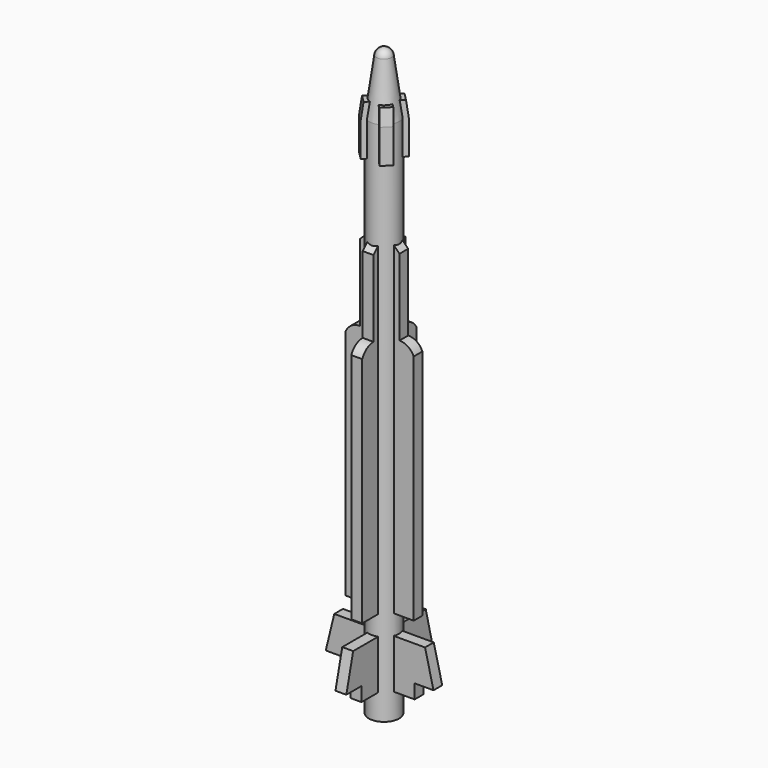
from build123d import *

# Parameters (mm, degrees)
F3_DEPTH     = 0.2
F6_DEPTH     = 0.2
F7_COUNT     = 4
F8_T4_DEPTH  = 1.685841494
F8_S5_R      = 0.5555555556
F8_T6_DEPTH  = 2
F8_T10_DEPTH = 1.685841494
F8_S11_R     = 0.5555555556
F8_T12_DEPTH = 2
F8_T16_DEPTH = 1.685841494
F8_S17_R     = 0.5555555556
F8_T18_DEPTH = 2
F8_T22_DEPTH = 1.685841494
F8_S23_R     = 0.5555555556
F8_T24_DEPTH = 2


# Not quite as in the source:
# - a fillet or chamfer that OpenCascade refuses, or shapes differently, is made with other operations: its cross-section is extruded or revolved along the edge and cut away or added
# - a feature names something its author has since deleted; it is built from what else it names


with BuildPart() as f1:
    # F0 (on Front) → F1 (revolve)
    with BuildSketch(Plane.XZ):
        with BuildLine():
            Line((0, 21.5277777778), (0, 0))
            Line((0, 0), (0.5555555556, 0))
            Line((0.5555555556, 0), (0.5555555556, 19.3055555556))
            Line((0.5555555556, 19.3055555556), (0.2793333296, 21.2847222222))
            ThreePointArc((0.2793333296, 21.2847222222), (0.185137187, 21.4585073218), (0, 21.5277777778))
        make_face()
    revolve(axis=Axis((0, 0, 10.7638888889), (0, 0, 1)))

    # F2 (on Front) → F3 (join, symmetric)
    with BuildSketch(Plane.XZ):
        with BuildLine():
            Line((0, 15.4166666667), (0, 3.4722222222))
            Line((0, 3.4722222222), (1.25, 3.4722222222))
            Line((1.25, 3.4722222222), (1.25, 12.0138888889))
            ThreePointArc((1.25, 12.0138888889), (1.0421485482, 12.2663478223), (0.7291666667, 12.3611111111))
            Line((0.7291666667, 12.3611111111), (0.7291666667, 15.4166666667))
            Line((0.7291666667, 15.4166666667), (0, 15.4166666667))
        make_face()
        Polygon((0, 2.7430555556), (0, 0.9375), (1.2847222222, 0.9375), (1.2847222222, 1.4583333333), (1.9791666667, 1.4583333333), (1.6666666667, 2.7430555556), align=None)
    extrude(amount=F3_DEPTH, both=True)

    # F5 (on face) → F6 (join, symmetric)
    with BuildSketch(Plane(origin=(0, 0, 0), x_dir=(0.7071067812, -0.7071067812, 0), z_dir=(-0.7071067812, -0.7071067812, 0))):
        Polygon((0, 19.3055555556), (0, 18.0555555556), (0.6944444444, 18.0555555556), (0.6944444444, 19.3055555556), (0.612062377, 19.8958333333), (0, 19.8958333333), align=None)
    extrude(amount=F6_DEPTH, both=True)

    # F7: F1 ×4 about axis
    f7_axis = Axis((0, 0, 0), (0, 0, 1))


with BuildPart() as f1_1:
    add(f1.part)
    for i in range(1, F7_COUNT):
        add(f1.part.rotate(f7_axis, i * 360 / F7_COUNT))

    # F8: chamfer of 0.25 on 4 edges, made by hand


with BuildPart() as f8_tool2:
    # F8_s3 → F8_t4 (new body)
    with BuildSketch(Plane.XZ.offset(0.842920747)):
        Polygon((-0.7291666667, 15.1666666667), (-0.4791666667, 15.4166666667), (-0.7291666667, 15.4166666667), align=None)
    extrude(amount=-F8_T4_DEPTH)

    # F8_s5 → F8_t6 (cut, symmetric)
    with BuildSketch(Plane.XY.offset(15.3)):
        Circle(F8_S5_R)
    extrude(amount=F8_T6_DEPTH, both=True, mode=Mode.SUBTRACT)


with BuildPart() as f1_2:
    add(f1_1.part)

    # F8_t1: cut F8_tool2
    add(f8_tool2.part, mode=Mode.SUBTRACT)


with BuildPart() as f8_tool8:
    # F8_s9 → F8_t10 (new body)
    with BuildSketch(Plane.YZ.offset(0.842920747)):
        Polygon((-0.7291666667, 15.1666666667), (-0.4791666667, 15.4166666667), (-0.7291666667, 15.4166666667), align=None)
    extrude(amount=-F8_T10_DEPTH)

    # F8_s11 → F8_t12 (cut, symmetric)
    with BuildSketch(Plane.XY.offset(15.3)):
        Circle(F8_S11_R)
    extrude(amount=F8_T12_DEPTH, both=True, mode=Mode.SUBTRACT)


with BuildPart() as f1_3:
    add(f1_2.part)

    # F8_t7: cut F8_tool8
    add(f8_tool8.part, mode=Mode.SUBTRACT)


with BuildPart() as f8_tool14:
    # F8_s15 → F8_t16 (new body)
    with BuildSketch(Plane.XZ.offset(-0.842920747)):
        Polygon((0.7291666667, 15.1666666667), (0.4791666667, 15.4166666667), (0.7291666667, 15.4166666667), align=None)
    extrude(amount=F8_T16_DEPTH)

    # F8_s17 → F8_t18 (cut, symmetric)
    with BuildSketch(Plane.XY.offset(15.3)):
        Circle(F8_S17_R)
    extrude(amount=F8_T18_DEPTH, both=True, mode=Mode.SUBTRACT)


with BuildPart() as f1_4:
    add(f1_3.part)

    # F8_t13: cut F8_tool14
    add(f8_tool14.part, mode=Mode.SUBTRACT)


with BuildPart() as f8_tool20:
    # F8_s21 → F8_t22 (new body)
    with BuildSketch(Plane.YZ.offset(-0.842920747)):
        Polygon((0.4791666667, 15.4166666667), (0.7291666667, 15.1666666667), (0.7291666667, 15.4166666667), align=None)
    extrude(amount=F8_T22_DEPTH)

    # F8_s23 → F8_t24 (cut, symmetric)
    with BuildSketch(Plane.XY.offset(15.3)):
        Circle(F8_S23_R)
    extrude(amount=F8_T24_DEPTH, both=True, mode=Mode.SUBTRACT)


with BuildPart() as f1_5:
    add(f1_4.part)

    # F8_t19: cut F8_tool20
    add(f8_tool20.part, mode=Mode.SUBTRACT)


solid = f1_5.part
